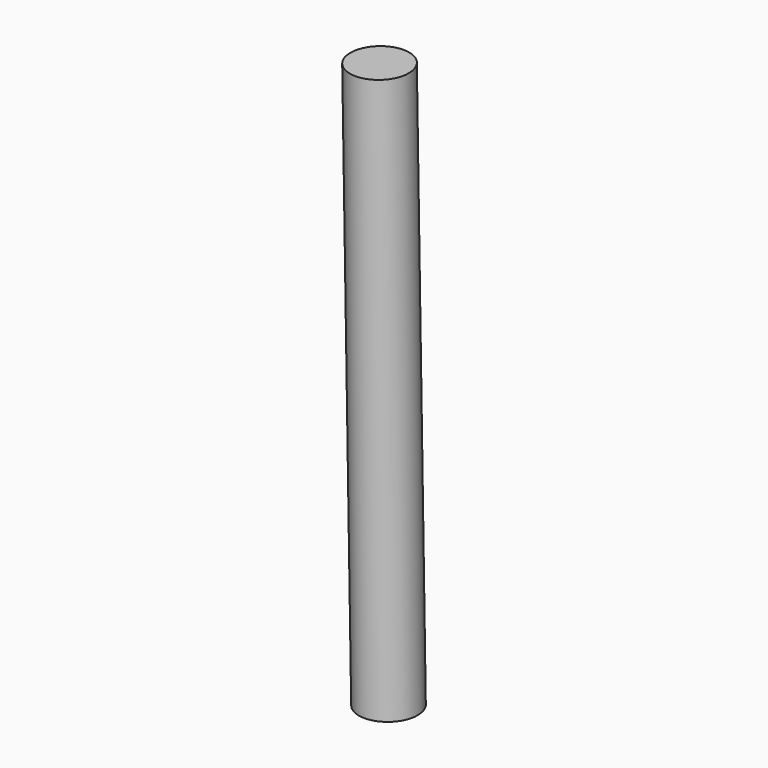
from build123d import *

# Parameters (mm, degrees)
F2_R = 50.8


with BuildPart() as f3:
    # F3: sweep along a path in F0
    with BuildLine(Plane.XZ) as f3_path:
        Line((136.979571281, 96.4017822322), (152.6, -882.7))
    # F2 (on face) → F3 (sweep)
    with BuildSketch(Plane(origin=(6.3074833784, 0, -395.3584327465), x_dir=(0.9998727619, 0, 0.0159518055), z_dir=(0.0159518055, 0, -0.9998727619))):
        with Locations((138.4999247355, 0)):
            Circle(F2_R)
    sweep(path=f3_path.line)


solid = f3.part
